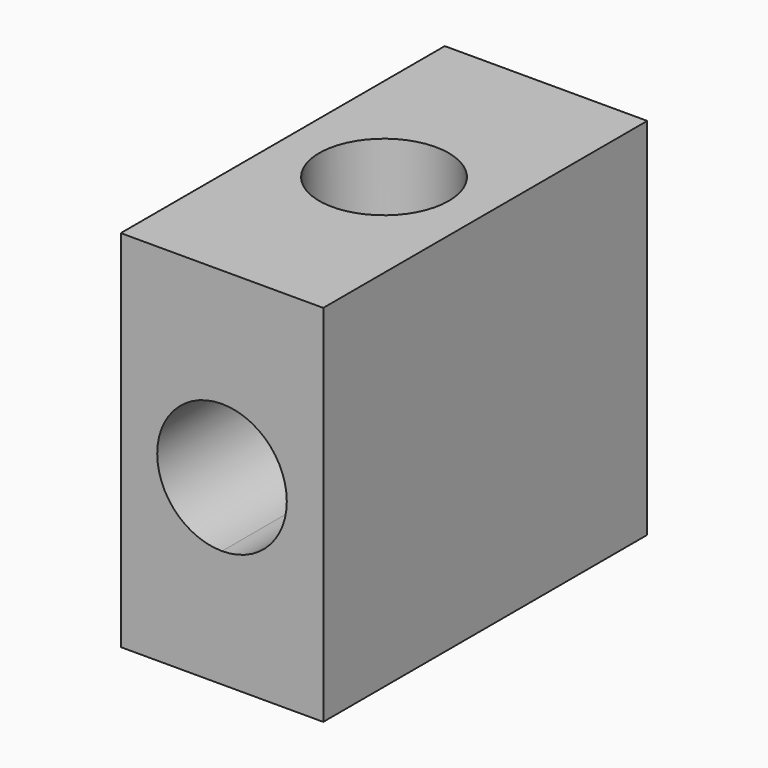
from build123d import *

# Parameters (mm, degrees)
F0_W     = 5
F0_H     = 10
F0_R     = 1.6
F1_DEPTH = 9
F3_DEPTH = 25


with BuildPart() as f1:
    # F0 (on Top) → F1 (new body)
    with BuildSketch(Plane.XY):
        Rectangle(F0_W, F0_H)
        Circle(F0_R, mode=Mode.SUBTRACT)
    extrude(amount=F1_DEPTH)

    # F2 (on face) → F3 (cut)
    with BuildSketch(Plane.XZ.offset(5)):
        with BuildLine():
            Line((0, 2.9), (0, 6.1))
            ThreePointArc((0, 6.1), (-1.6, 4.5), (0, 2.9))
        make_face()
        with BuildLine():
            ThreePointArc((1.6, 4.5), (1.131371, 5.631371), (0, 6.1))
            Line((0, 6.1), (0, 2.9))
            ThreePointArc((0, 2.9), (1.131371, 3.368629), (1.6, 4.5))
        make_face()
    extrude(amount=-F3_DEPTH, mode=Mode.SUBTRACT)


solid = f1.part
